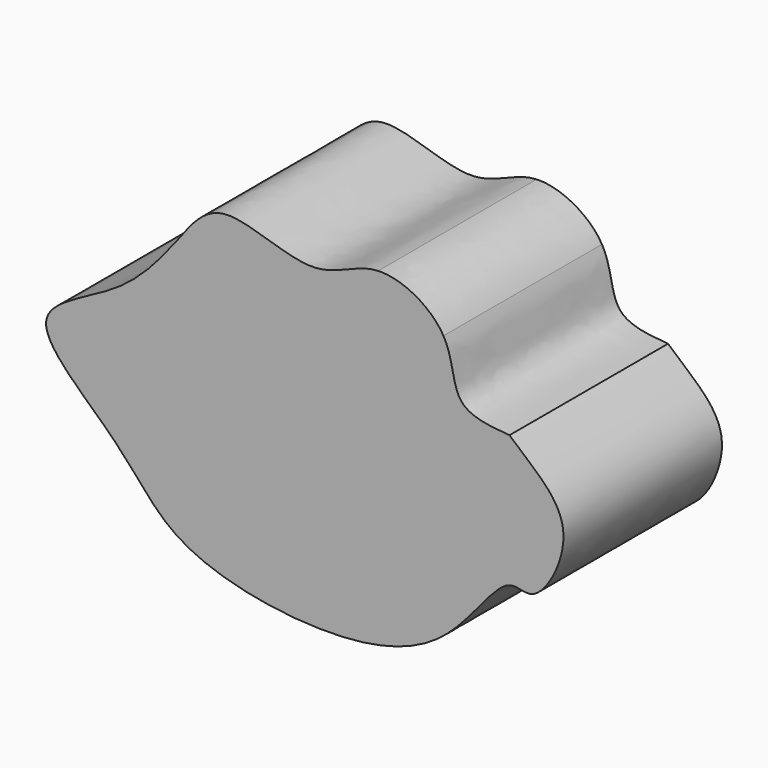
from build123d import *

# Parameters (mm, degrees)
F1_DEPTH = 76.2


with BuildPart() as f1:
    # F0 (on Front) → F1 (new body)
    with BuildSketch(Plane.XZ):
        with BuildLine():
            add(Edge.make_bspline(
                [(24.9060709029, 46.9583794475), (16.1727104769, 46.5660775171), (1.2227384931, 33.0502935537), (-35.8883926105, 54.3429364547), (-46.7549393931, 39.6552097469), (-51.563370645, 33.1559118986)],
                knots=[0.4774119485, 0.4774119485, 0.4774119485, 0.4774119485, 0.6465909332, 0.8436169985, 1, 1, 1, 1], degree=3))
            add(Edge.make_bspline(
                [(-51.563370645, 33.1559118986), (-58.6568476295, 24.0181643446), (-72.471094018, 6.22278749), (-117.9873713114, -9.4862487022), (-72.4665303899, -43.6990176605), (-55.5397089554, -72.7251306361), (0.6684223402, -85.0543128637), (51.5855769231, -76.8486488178), (73.1719149378, -37.628342201), (86.0831026078, -48.2844127901), (104.7431469221, -13.2655589993), (84.3400045117, -0.34321211), (75.436629355, 7.7559118986)],
                knots=[0, 0, 0, 0, 0.0857700941, 0.1670336304, 0.2582623164, 0.3440324105, 0.4483871845, 0.551280309, 0.6370504031, 0.68014386, 0.7556252198, 0.8376020816, 0.8376020816, 0.8376020816, 0.8376020816], degree=3))
            add(Edge.make_bspline(
                [(75.436629355, 7.7559118986), (67.9168082181, 8.3604978714), (52.5428657153, 9.5965472156), (54.062471008, 26.185396649), (50.036629355, 33.1559118986)],
                knots=[0, 0, 0, 0, 0.1463166779, 0.2991379918, 0.2991379918, 0.2991379918, 0.2991379918], degree=3))
            add(Edge.make_bspline(
                [(50.036629355, 33.1559118986), (42.3076569703, 39.3659677496), (33.6068639366, 43.1621735986), (24.9060709029, 46.9583794475)],
                knots=[0.9233721757, 0.9233721757, 0.9233721757, 0.9233721757, 1, 1, 1, 1], degree=3))
        make_face()
        with BuildLine():
            add(Edge.make_bspline(
                [(50.036629355, 33.1559118986), (45.3402771089, 41.2873780041), (34.1089321341, 47.3717713207), (24.9060709029, 46.9583794475)],
                knots=[0.2991379918, 0.2991379918, 0.2991379918, 0.2991379918, 0.4774119485, 0.4774119485, 0.4774119485, 0.4774119485], degree=3))
            add(Edge.make_bspline(
                [(50.036629355, 33.1559118986), (42.3076569703, 39.3659677496), (33.6068639366, 43.1621735986), (24.9060709029, 46.9583794475)],
                knots=[0.9233721757, 0.9233721757, 0.9233721757, 0.9233721757, 1, 1, 1, 1], degree=3))
        make_face()
    extrude(amount=F1_DEPTH)


solid = f1.part
